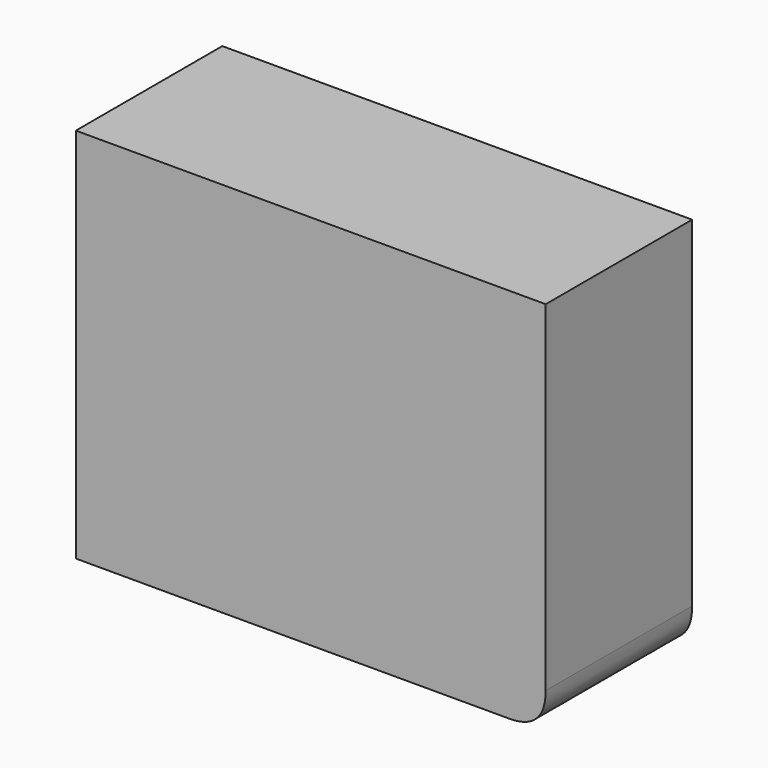
from build123d import *

# Parameters (mm, degrees)
F0_W        = 64.1731321812
F0_H        = 51.4541268349
F1_DEPTH    = 25
F2_T1_DEPTH = 50


# Not quite as in the source:
# - a fillet or chamfer that OpenCascade refuses, or shapes differently, is made with other operations: its cross-section is extruded or revolved along the edge and cut away or added


with BuildPart() as f1:
    # F0 (on Front) → F1 (new body)
    with BuildSketch(Plane.XZ):
        with Locations((-144.389539957, 48.7079843879)):
            Rectangle(F0_W, F0_H)
    extrude(amount=F1_DEPTH)

    # F2: fillet of radius 5 on 1 edges, made by hand

    # F2_s2 → F2_t1 (cut)
    with BuildSketch(Plane.XZ.offset(-12.5)):
        with BuildLine():
            add(Edge.make_bspline(
                [(-117.3029738665, 22.9809209704), (-112.3029738665, 22.9809209704), (-112.3029738665, 27.9809209704)],
                knots=[0, 0, 0, 1, 1, 1], degree=2, weights=[1, 1, 1]))
            Line((-112.3029738665, 27.9809209704), (-112.3029738665, 22.9809209704))
            Line((-112.3029738665, 22.9809209704), (-117.3029738665, 22.9809209704))
        make_face()
    extrude(amount=F2_T1_DEPTH, mode=Mode.SUBTRACT)


solid = f1.part
